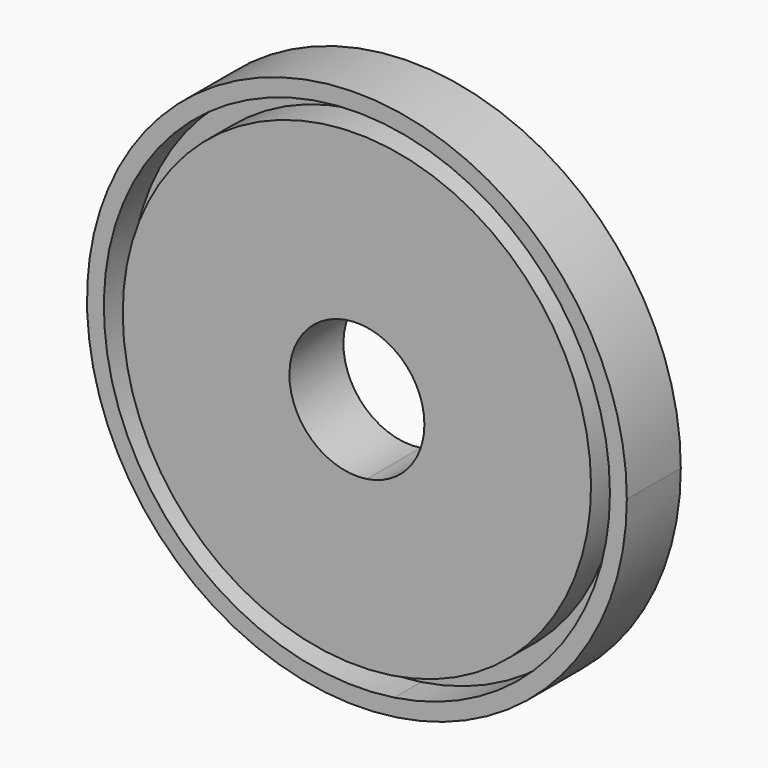
from build123d import *

# Parameters (mm, degrees)
F1_DEPTH = 12.7
F2_DEPTH = 6.35


with BuildPart() as f1:
    # F0 (on Front) → F1 (new body)
    with BuildSketch(Plane.XZ):
        with BuildLine():
            ThreePointArc((7.4964542451, -50.2438371719), (38.480253869, -33.1648920121), (50.8, 0))
            ThreePointArc((50.8, 0), (-38.480253869, 33.1648920121), (7.4964542451, -50.2438371719))
        make_face()
        with BuildLine():
            ThreePointArc((47.625, 0), (36.0752380022, -31.0920862614), (7.0279258548, -47.1035973486))
            ThreePointArc((7.0279258548, -47.1035973486), (-36.0752380022, 31.0920862614), (47.625, 0))
        make_face(mode=Mode.SUBTRACT)
    extrude(amount=F1_DEPTH)

    # F0 (on Front) → F2 (join)
    with BuildSketch(Plane.XZ):
        with BuildLine():
            ThreePointArc((47.625, 0), (-36.0752380022, 31.0920862614), (7.0279258548, -47.1035973486))
            ThreePointArc((7.0279258548, -47.1035973486), (36.0752380022, -31.0920862614), (47.625, 0))
        make_face()
        with BuildLine():
            ThreePointArc((44.069, 0), (33.3816202314, -28.7705438205), (6.5031740576, -43.5865287466))
            ThreePointArc((6.5031740576, -43.5865287466), (-33.3816202314, 28.7705438205), (44.069, 0))
        make_face(mode=Mode.SUBTRACT)
    extrude(amount=F2_DEPTH)


with BuildPart() as f1b:
    # F0 (on Front) → F1, piece 2 (new body)
    with BuildSketch(Plane.XZ):
        with BuildLine():
            ThreePointArc((44.069, 0), (-33.3816202314, 28.7705438205), (6.5031740576, -43.5865287466))
            ThreePointArc((6.5031740576, -43.5865287466), (33.3816202314, -28.7705438205), (44.069, 0))
        make_face()
        with BuildLine():
            ThreePointArc((12.7, 0), (9.6200634673, -8.291223003), (1.8741135613, -12.560959293))
            ThreePointArc((1.8741135613, -12.560959293), (-9.6200634673, 8.291223003), (12.7, 0))
        make_face(mode=Mode.SUBTRACT)
    extrude(amount=F1_DEPTH)


solid = Compound([f1.part, f1b.part])
